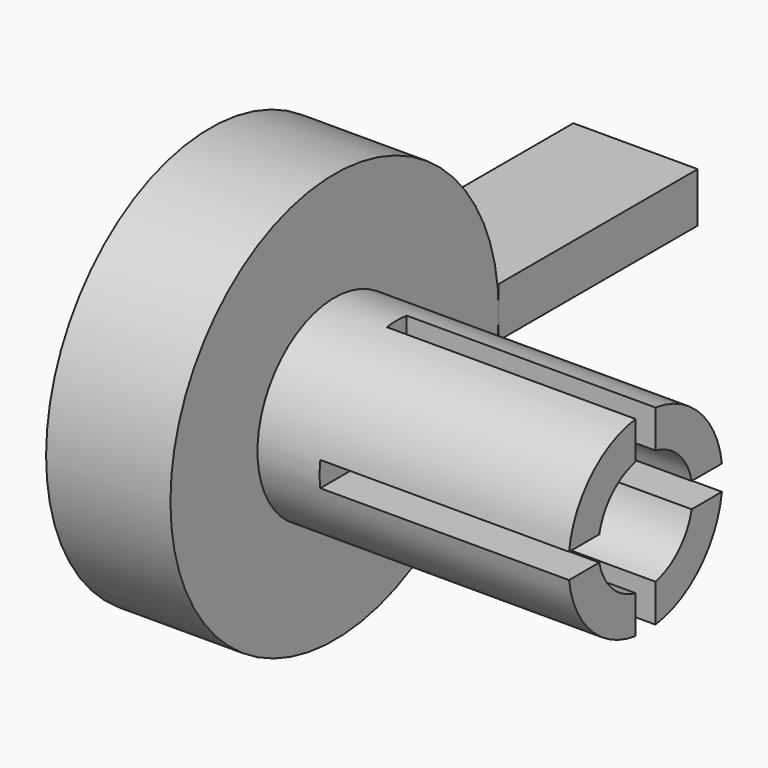
from build123d import *

# Parameters (mm, degrees)
F0_W     = 25
F0_H     = 7.75
F2_W     = 2
F2_H     = 2
F3_DEPTH = 20
F4_R     = 4.5
F4_R_2   = 1.5
F5_DEPTH = 5
F6_DEPTH = 25
F7_W     = 10
F7_H     = 20
F8_DEPTH = 2
F9_DEPTH = 2


# Not quite as in the source:
# - a feature names something its author has since deleted; it is built from what else it names


with BuildPart() as f1:
    # F0 (on Top) → F1 (revolve)
    with BuildSketch(Plane.XY):
        Polygon((-10, 0), (0, 0), (0, 7.75), (0, 16.5), (-10, 16.5), align=None)
        with Locations((12.5, 3.875)):
            Rectangle(F0_W, F0_H)
    revolve(axis=Axis((12.5, 0, 0), (1, 0, 0)))

    # F2 (on face) → F3 (cut)
    with BuildSketch(Plane.YZ.offset(25)):
        with BuildLine():
            ThreePointArc((4.6435439053, 1), (4.7233109971, 0.502825243), (4.75, 0))
            ThreePointArc((4.75, 0), (4.7233109971, -0.502825243), (4.6435439053, -1))
            Line((4.6435439053, -1), (7.6852130745, -1))
            ThreePointArc((7.6852130745, -1), (7.7337863084, -0.5010482376), (7.75, 0))
            ThreePointArc((7.75, 0), (7.7337863084, 0.5010482376), (7.6852130745, 1))
            Line((7.6852130745, 1), (4.6435439053, 1))
        make_face()
        with BuildLine():
            Line((10.7483885819, 1), (7.6852130745, 1))
            ThreePointArc((7.6852130745, 1), (7.7337863084, 0.5010482376), (7.75, 0))
            ThreePointArc((7.75, 0), (7.7337863084, -0.5010482376), (7.6852130745, -1))
            Line((7.6852130745, -1), (10.7483885819, -1))
            Line((10.7483885819, -1), (10.7483885819, 1))
        make_face()
        with BuildLine():
            ThreePointArc((4.6435439053, -1), (4.7233109971, -0.502825243), (4.75, 0))
            ThreePointArc((4.75, 0), (4.7233109971, 0.502825243), (4.6435439053, 1))
            Line((4.6435439053, 1), (1, 1))
            Line((1, 1), (1, -1))
            Line((1, -1), (4.6435439053, -1))
        make_face()
        with BuildLine():
            Line((1, 1), (1, 4.6435439053))
            ThreePointArc((1, 4.6435439053), (0, 4.75), (-1, 4.6435439053))
            Line((-1, 4.6435439053), (-1, 1))
            Line((-1, 1), (1, 1))
        make_face()
        with BuildLine():
            ThreePointArc((-1, 4.6435439053), (0, 4.75), (1, 4.6435439053))
            Line((1, 4.6435439053), (1, 7.6852130745))
            ThreePointArc((1, 7.6852130745), (0, 7.75), (-1, 7.6852130745))
            Line((-1, 7.6852130745), (-1, 4.6435439053))
        make_face()
        with BuildLine():
            ThreePointArc((-1, 7.6852130745), (0, 7.75), (1, 7.6852130745))
            Line((1, 7.6852130745), (1, 10.1087059955))
            Line((1, 10.1087059955), (-1, 10.1087059955))
            Line((-1, 10.1087059955), (-1, 7.6852130745))
        make_face()
        Rectangle(F2_W, F2_H)
        with BuildLine():
            ThreePointArc((-1, -4.6435439053), (0, -4.75), (1, -4.6435439053))
            Line((1, -4.6435439053), (1, -1))
            Line((1, -1), (-1, -1))
            Line((-1, -1), (-1, -4.6435439053))
        make_face()
        with BuildLine():
            Line((1, -7.6852130745), (1, -4.6435439053))
            ThreePointArc((1, -4.6435439053), (0, -4.75), (-1, -4.6435439053))
            Line((-1, -4.6435439053), (-1, -7.6852130745))
            ThreePointArc((-1, -7.6852130745), (0, -7.75), (1, -7.6852130745))
        make_face()
        with BuildLine():
            Line((1, -10.1087059955), (1, -7.6852130745))
            ThreePointArc((1, -7.6852130745), (0, -7.75), (-1, -7.6852130745))
            Line((-1, -7.6852130745), (-1, -10.1087059955))
            Line((-1, -10.1087059955), (1, -10.1087059955))
        make_face()
        with BuildLine():
            Line((-1, -1), (-1, 1))
            Line((-1, 1), (-4.6435439053, 1))
            ThreePointArc((-4.6435439053, 1), (-4.75, 0), (-4.6435439053, -1))
            Line((-4.6435439053, -1), (-1, -1))
        make_face()
        with BuildLine():
            ThreePointArc((-4.6435439053, -1), (-4.75, 0), (-4.6435439053, 1))
            Line((-4.6435439053, 1), (-7.6852130745, 1))
            ThreePointArc((-7.6852130745, 1), (-7.75, 0), (-7.6852130745, -1))
            Line((-7.6852130745, -1), (-4.6435439053, -1))
        make_face()
        with BuildLine():
            ThreePointArc((-7.6852130745, -1), (-7.75, 0), (-7.6852130745, 1))
            Line((-7.6852130745, 1), (-10.7483885819, 1))
            Line((-10.7483885819, 1), (-10.7483885819, -1))
            Line((-10.7483885819, -1), (-7.6852130745, -1))
        make_face()
        with BuildLine():
            Line((-1, 1), (-1, 4.6435439053))
            ThreePointArc((-1, 4.6435439053), (-3.3587572106, 3.3587572106), (-4.6435439053, 1))
            Line((-4.6435439053, 1), (-1, 1))
        make_face()
        with BuildLine():
            ThreePointArc((-4.6435439053, -1), (-3.3587572106, -3.3587572106), (-1, -4.6435439053))
            Line((-1, -4.6435439053), (-1, -1))
            Line((-1, -1), (-4.6435439053, -1))
        make_face()
        with BuildLine():
            ThreePointArc((1, -4.6435439053), (3.3587572106, -3.3587572106), (4.6435439053, -1))
            Line((4.6435439053, -1), (1, -1))
            Line((1, -1), (1, -4.6435439053))
        make_face()
        with BuildLine():
            Line((1, 1), (4.6435439053, 1))
            ThreePointArc((4.6435439053, 1), (3.3587572106, 3.3587572106), (1, 4.6435439053))
            Line((1, 4.6435439053), (1, 1))
        make_face()
    extrude(amount=-F3_DEPTH, mode=Mode.SUBTRACT)

    # F4 (on face) → F5 (cut)
    with BuildSketch(Plane(origin=(-10, 0, 0), x_dir=(0, -1, 0), z_dir=(-1, 0, 0))):
        Circle(F4_R)
        Circle(F4_R_2, mode=Mode.SUBTRACT)
    extrude(amount=-F5_DEPTH, mode=Mode.SUBTRACT)

    # F6 (cut): a face of the model
    f6_faces = [f1.faces().sort_by_distance(p)[0] for p in [
        (-10, 0, 0),
    ]]
    extrude(f6_faces, amount=-F6_DEPTH, mode=Mode.SUBTRACT)

    # F7 (on Top) → F8 (join)
    with BuildSketch(Plane.XY):
        with Locations((-5, 26.5)):
            Rectangle(F7_W, F7_H)
    extrude(amount=F8_DEPTH)

    # F7 (on Top) → F9 (join)
    with BuildSketch(Plane.XY):
        with Locations((-5, 26.5)):
            Rectangle(F7_W, F7_H)
    extrude(amount=-F9_DEPTH)


solid = f1.part
